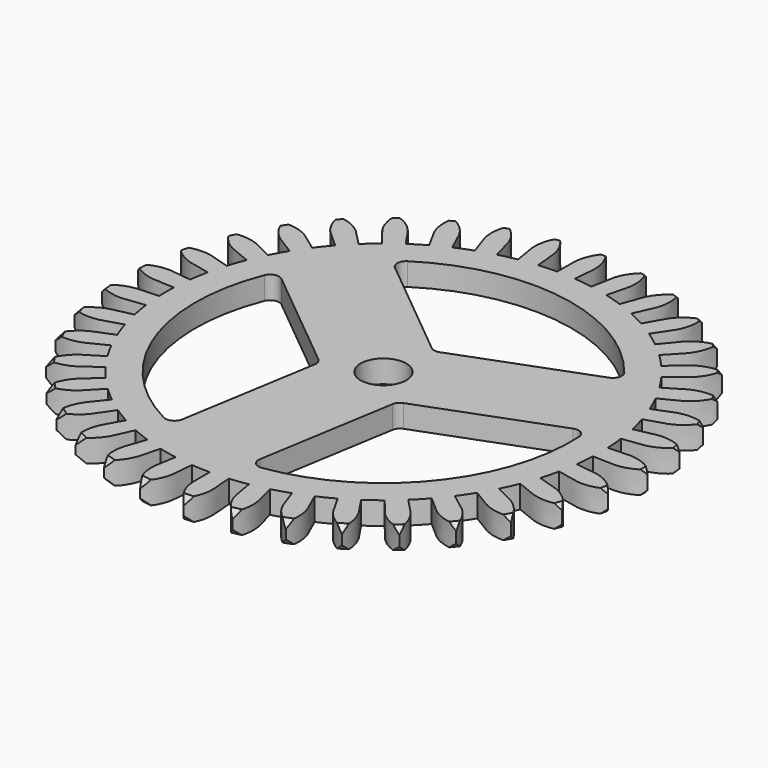
from build123d import *

# Parameters (mm, degrees)
F1_DEPTH = 2.5
F2_COUNT = 38
F2_ANGLE = 359.973
F3_R     = 2.515
F4_DEPTH = 2.5010001


# Not quite as in the source:
# - ends of sketch curves that miss each other by under 0.0002 mm in the source are joined


with BuildPart() as f1:
    # F0 (on Top) → F1 (new body)
    with BuildSketch(Plane.XY):
        with BuildLine():
            Line((14.1996744578, 1.0151064721), (18.0441680012, 23.4027091839))
            ThreePointArc((18.0441680012, 23.4027091839), (17.0381281371, 23.5535648399), (16.0265928019, 23.661592164))
            add(Edge.make_bspline(
                [(16.0265928019, 23.661592164), (16.083143395, 24.3321523545), (16.1696731688, 25.3581378284), (16.2195672424, 25.9021061443), (16.2190815269, 26.184112899), (16.1974303413, 26.7229190909), (16.0395989717, 27.4627632881), (15.7392035716, 28.1736485112), (15.4624982931, 28.6223385091), (15.3044857432, 28.831404832), (15.232194, 28.927054)],
                knots=[0.0004962398, 0.0004962398, 0.0004962398, 0.0004962398, 0.2089847892, 0.3197775881, 0.4000126581, 0.5133023611, 0.6520840168, 0.7908656467, 0.9043197077, 1, 1, 1, 1], degree=3))
            add(Edge.make_bspline(
                [(13.9941067747, 23.7484608841), (13.9934095521, 24.4604460167), (13.9923548553, 25.5445332098), (13.9970761199, 26.1076252879), (14.027686201, 26.3872952), (14.1082367384, 26.9205369872), (14.3541265235, 27.6465869132), (14.721906747, 28.3320011048), (15.0620982821, 28.7287030736), (15.232194, 28.927054)],
                knots=[0.0005711622, 0.0005711622, 0.0005711622, 0.0005711622, 0.2292078439, 0.3490311048, 0.4344432416, 0.5555548274, 0.7037031584, 0.8518516225, 1, 1, 1, 1], degree=3))
            add(Edge.make_bspline(
                [(13.994112, 23.743125), (13.9941102582, 23.7449036294), (13.9941085164, 23.7466822589), (13.9941067747, 23.7484608841)],
                knots=[0, 0, 0, 0, 0.0005711622, 0.0005711622, 0.0005711622, 0.0005711622], degree=3))
            Line((13.994112, 23.743125), (13.9881880901, 1.0331609575))
            Line((13.9881880901, 1.0331609575), (13.987862, -0.218339))
            Line((13.987862, -0.218339), (14.1996744578, 1.0151064721))
        make_face()
    extrude(amount=F1_DEPTH)

    # F2: F1 ×38 about axis
    f2_axis = Axis((13.987862, -0.218339, 1.25), (0, 0, -1))


with BuildPart() as f1_1:
    add(f1.part)
    for i in range(1, F2_COUNT):
        add(f1.part.rotate(f2_axis, i * F2_ANGLE / (F2_COUNT - 1)))

    # F3 (on face) → F4 (cut, through all)
    with BuildSketch(Plane.XY.offset(2.5)):
        with Locations((13.9876825093, -0.2212404145)):
            Circle(F3_R)
        with BuildLine():
            ThreePointArc((-3.7359316465, 7.8605050327), (-4.6200512351, 8.0559674507), (-5.2995458525, 7.4575026909))
            ThreePointArc((-5.2995458525, 7.4575026909), (-5.4427054418, -7.5301594611), (4.5427868627, -18.7078360931))
            ThreePointArc((4.5427868627, -18.7078360931), (5.4482524129, -18.7101035156), (5.9843652019, -17.9804076329))
            Line((5.9843652019, -17.9804076329), (8.4896911133, -2.8235644394))
            ThreePointArc((8.4896911133, -2.8235644394), (8.4390503485, -2.308409409), (8.1376166446, -1.8875924481))
            Line((8.1376166446, -1.8875924481), (-3.7359316465, 7.8605050327))
        make_face()
        with BuildLine():
            Line((2.6094512193, 15.5894193088), (14.4829994965, 5.8413218394))
            ThreePointArc((14.4829994965, 5.8413218394), (14.9544572222, 5.6276005129), (15.4696122526, 5.6782412776))
            Line((15.4696122526, 5.6782412776), (29.8484864383, 11.0869869841))
            ThreePointArc((29.8484864383, 11.0869869841), (30.4598216522, 11.7549257993), (30.2812832749, 12.6426177799))
            ThreePointArc((30.2812832749, 12.6426177799), (17.3731669162, 20.2604286798), (2.7002688639, 17.2015770028))
            ThreePointArc((2.7002688639, 17.2015770028), (2.2455724424, 16.4185545453), (2.6094512193, 15.5894193088))
        make_face()
        with BuildLine():
            Line((33.3692311252, 1.7272670711), (18.9903569395, -3.6814786354))
            ThreePointArc((18.9903569395, -3.6814786354), (18.5695399786, -3.9829123393), (18.3558186521, -4.4543700649))
            Line((18.3558186521, -4.4543700649), (15.8504927437, -19.6112132408))
            ThreePointArc((15.8504927437, -19.6112132408), (16.1232771189, -20.4746144739), (16.9813101135, -20.7638416939))
            ThreePointArc((16.9813101135, -20.7638416939), (30.0325860533, -13.3939904622), (34.7199918208, 0.8425378368))
            ThreePointArc((34.7199918208, 0.8425378368), (34.2692226916, 1.6278277175), (33.3692311252, 1.7272670711))
        make_face()
    extrude(amount=-F4_DEPTH, mode=Mode.SUBTRACT)

    # F5 (on Front) → F6 (revolve, cut)
    with BuildSketch(Plane.XZ):
        Polygon((-14.5786680256, 0), (-15.8286680256, 1.25), (-14.5786680256, 2.5), (-17.6396388561, 2.5), (-17.6396388561, 0), align=None)
    revolve(axis=Axis((14.0405687309, 0, 3.2905454282), (0, 0, 1)), mode=Mode.SUBTRACT)


solid = f1_1.part
